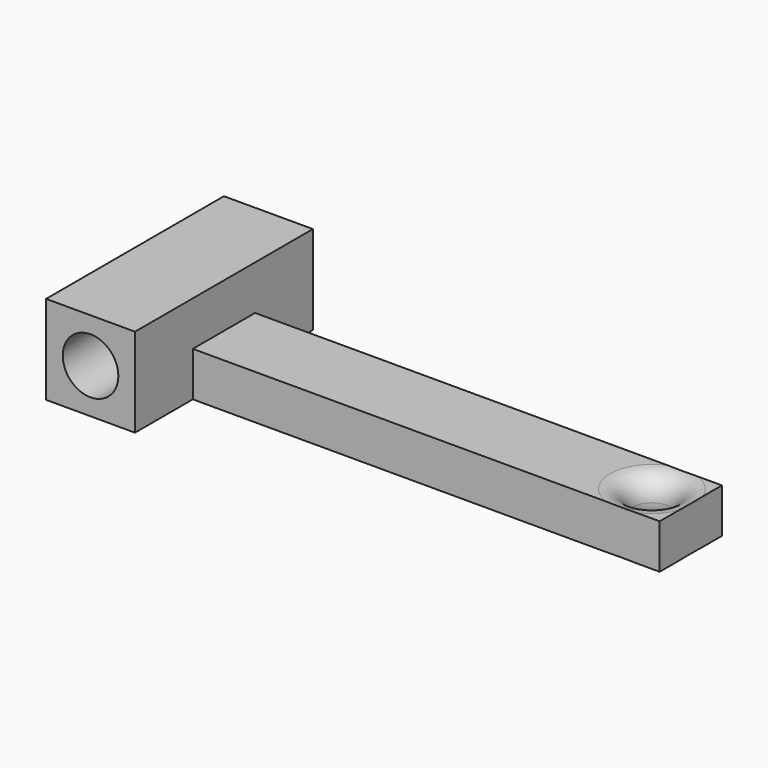
from build123d import *

# Parameters (mm, degrees)
F1_DEPTH = 8
F0_W     = 42
F0_H     = 7
F0_R     = 1.75
F2_DEPTH = 4
F4_R     = 2.5
F5_DEPTH = 20.001


# Not quite as in the source:
# - a fillet or chamfer that OpenCascade refuses, or shapes differently, is made with other operations: its cross-section is extruded or revolved along the edge and cut away or added


with BuildPart() as f1:
    # F0 (on Top) → F1 (new body)
    with BuildSketch(Plane.XY):
        Polygon((0, -6.5), (0, 0), (0, 7), (0, 13.5), (-8, 13.5), (-8, -6.5), align=None)
    extrude(amount=F1_DEPTH)

    # F0 (on Top) → F2 (join)
    with BuildSketch(Plane.XY):
        with Locations((21, 3.5)):
            Rectangle(F0_W, F0_H)
        with Locations((38.5, 3.5)):
            Circle(F0_R, mode=Mode.SUBTRACT)
    extrude(amount=F2_DEPTH)

    # F3: fillet of radius 2 on 2 edges, made by hand

    # F3_s1 → F3_t2 (revolve, cut)
    with BuildSketch(Plane.XZ.offset(-3.5)):
        with BuildLine():
            ThreePointArc((42.25, 4), (40.8357864376, 3.4142135624), (40.25, 2))
            Line((40.25, 2), (40.25, 4))
            Line((40.25, 4), (42.25, 4))
        make_face()
    revolve(axis=Axis((38.5, 3.5, 4), (0, 0, 1)), mode=Mode.SUBTRACT)

    # F3_s3 → F3_t4 (revolve, cut)
    with BuildSketch(Plane.XZ.offset(-3.5)):
        with BuildLine():
            ThreePointArc((42.25, 0), (40.8357864376, 0.5857864376), (40.25, 2))
            Line((40.25, 2), (40.25, 0))
            Line((40.25, 0), (42.25, 0))
        make_face()
    revolve(axis=Axis((38.5, 3.5, 0), (0, 0, 1)), mode=Mode.SUBTRACT)

    # F4 (on face) → F5 (cut, through all)
    with BuildSketch(Plane.XZ.offset(6.5)):
        with Locations((-4, 4)):
            Circle(F4_R)
    extrude(amount=-F5_DEPTH, mode=Mode.SUBTRACT)


solid = f1.part
